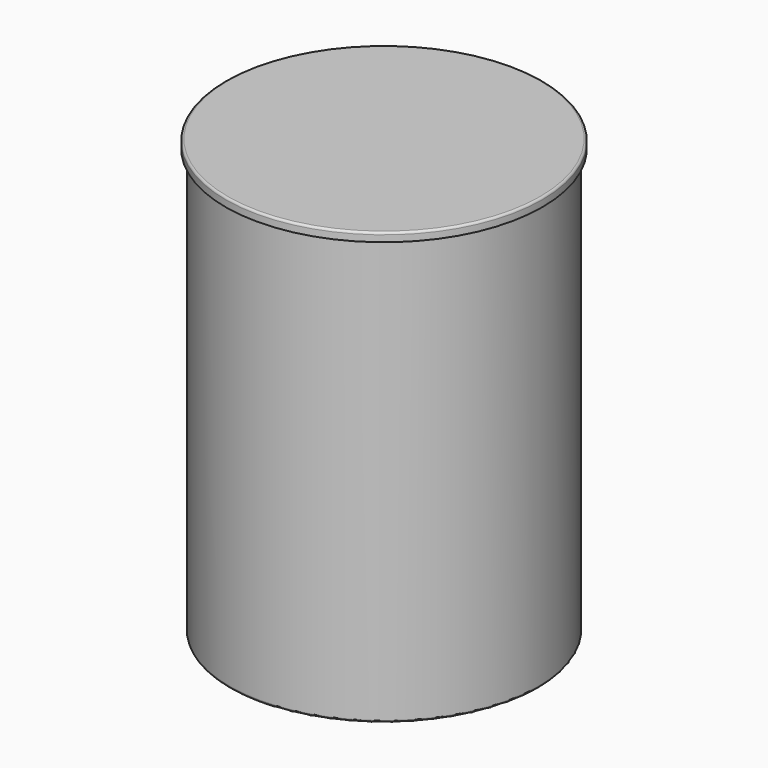
from build123d import *

# Parameters (mm, degrees)
F0_R     = 35.5
F0_R_2   = 34.5
F1_DEPTH = 100
F2_R     = 36.5
F3_DEPTH = 2
F4_R     = 0.49999


# Not quite as in the source:
# - a fillet or chamfer is up to 0.001 mm smaller than in the source, because OpenCascade refuses the exact size


with BuildPart() as f1:
    # F0 (on Top) → F1 (new body)
    with BuildSketch(Plane.XY):
        Circle(F0_R)
        Circle(F0_R_2, mode=Mode.SUBTRACT)
    extrude(amount=F1_DEPTH)

    # F2 (on face) → F3 (join)
    with BuildSketch(Plane.XY.offset(100)):
        Circle(F2_R)
    extrude(amount=-F3_DEPTH)

    # F4 (radius 0.5 in the source; OpenCascade refuses exactly that, so slightly less here)
    f4_edges = [f1.edges().sort_by_distance(p)[0] for p in [
        (-35.5, 0, 0),
        (-34.5, 0, 0),
        (-36.5, 0, 100),
    ]]
    fillet(f4_edges, radius=F4_R)


solid = f1.part
